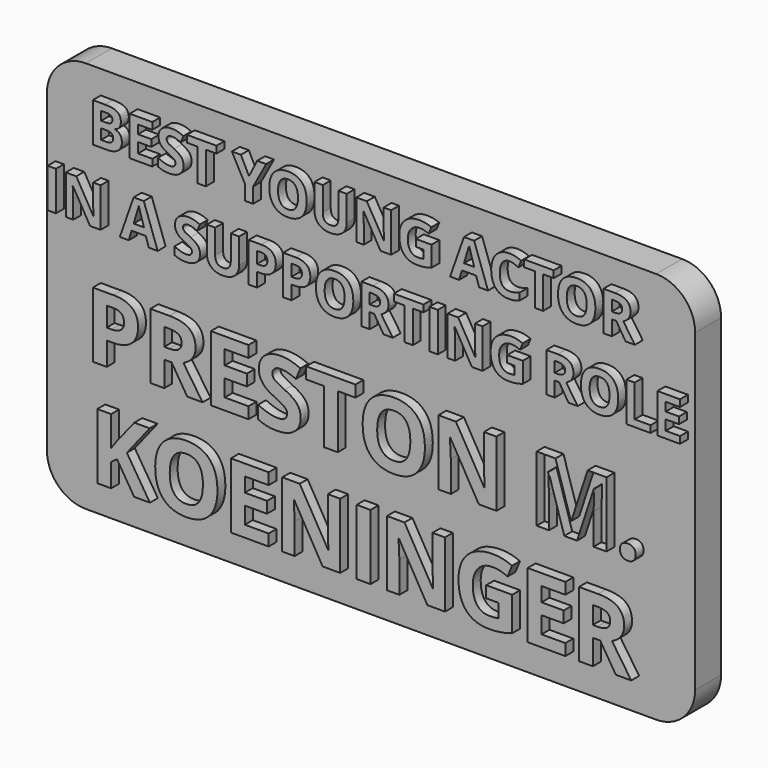
from build123d import *

# Parameters (mm, degrees)
F0_W           = 74
F0_H           = 47
F0_W_2         = 54
F0_H_2         = 27
F0_W_3         = 12.5
F0_H_3         = 6.5
F1_DEPTH       = 12
F2_W           = 54
F2_H           = 27
F3_DEPTH       = 32
F4_W           = 12.5
F4_H           = 6.5
F5_DEPTH       = 1
F7_R           = 3.556
F8_R           = 1.524
F9_R           = 0.762
F10_T          = -2.5
F6_TEXT_SIZE   = 4.2333333333
F6_TEXT_SIZE_2 = 7.0555555556
F11_DEPTH      = 0.762
F12_W          = 81.8964131176
F12_H          = 49.3911341764
F13_DEPTH      = 23.501
F13_DEPTH_BACK = 23.501
F14_W          = 63.7431629002
F14_H          = 29.3685784563
F15_DEPTH      = 30.2390001


# Not quite as in the source:
# - Text() gives the source's letters only with a copy of the font that has no kerning and outlines rounded to 1/6400 em; it was checked with that copy


with BuildPart() as f1:
    # F0 (on Top) → F1 (new body)
    with BuildSketch(Plane.XY):
        Rectangle(F0_W, F0_H)
        Rectangle(F0_W_2, F0_H_2, mode=Mode.SUBTRACT)
        Rectangle(F0_W_2, F0_H_2)
        Rectangle(F0_W_3, F0_H_3, mode=Mode.SUBTRACT)
        Rectangle(F0_W_3, F0_H_3)
    extrude(amount=F1_DEPTH)

    # F2 (on face) → F3 (join)
    with BuildSketch(Plane.XY.offset(12)):
        Rectangle(F2_W, F2_H)
    extrude(amount=F3_DEPTH)

    # F4 (on face) → F5 (cut)
    with BuildSketch(Plane.XY.offset(44)):
        Rectangle(F4_W, F4_H)
    extrude(amount=-F5_DEPTH, mode=Mode.SUBTRACT)

    # F7
    f7_edges = [f1.edges().sort_by_distance(p)[0] for p in [
        (-37, -23.5, 6),
        (37, -23.5, 6),
        (37, 23.5, 6),
        (-37, 23.5, 6),
    ]]
    fillet(f7_edges, radius=F7_R)

    # F8
    f8_edges = [f1.edges().sort_by_distance(p)[0] for p in [
        (-27, -13.5, 28),
        (27, -13.5, 28),
        (27, 13.5, 28),
        (-27, 13.5, 28),
    ]]
    fillet(f8_edges, radius=F8_R)

    # F9
    f9_edges = [f1.edges().sort_by_distance(p)[0] for p in [
        (0, -13.5, 44),
        (0, -23.5, 12),
    ]]
    fillet(f9_edges, radius=F9_R)

    # F10
    f10_openings = [f1.faces().sort_by_distance(p)[0] for p in [
        (0, 0, 0),
    ]]
    offset(amount=F10_T, openings=f10_openings, kind=Kind.INTERSECTION)

    # F6 (on face) → F11 (join)
    with BuildSketch(Plane.XZ.offset(13.5)):
        with Locations((-21.2123072917, 37.904)):
            Text('BEST YOUNG ACTOR', F6_TEXT_SIZE, font='Open Sans', font_style=FontStyle.BOLD, text_align=(TextAlign.LEFT, TextAlign.BOTTOM))
        with Locations((-24.6938932292, 32.316)):
            Text('IN A SUPPORTING ROLE', F6_TEXT_SIZE, font='Open Sans', font_style=FontStyle.BOLD, text_align=(TextAlign.LEFT, TextAlign.BOTTOM))
        with Locations((-21.4571571181, 23.172)):
            Text('PRESTON M.', F6_TEXT_SIZE_2, font='Open Sans', font_style=FontStyle.BOLD, text_align=(TextAlign.LEFT, TextAlign.BOTTOM))
        with Locations((-21.1176085069, 15.044)):
            Text('KOENINGER', F6_TEXT_SIZE_2, font='Open Sans', font_style=FontStyle.BOLD, text_align=(TextAlign.LEFT, TextAlign.BOTTOM))
    extrude(amount=F11_DEPTH)

    # F12 (on Front) → F13 (cut, two sides)
    with BuildSketch(Plane.XZ) as f13_sk:
        with Locations((0.2854410559, 21.6889909934)):
            Rectangle(F12_W, F12_H)
        with BuildLine():
            ThreePointArc((-24.976, 39.738), (-24.0973203436, 41.8593203436), (-21.976, 42.738))
            Line((-21.976, 42.738), (21.976, 42.738))
            ThreePointArc((21.976, 42.738), (24.0973203436, 41.8593203436), (24.976, 39.738))
            Line((24.976, 39.738), (24.976, 15.5))
            ThreePointArc((24.976, 15.5), (24.0973203436, 13.3786796564), (21.976, 12.5))
            Line((21.976, 12.5), (-21.976, 12.5))
            ThreePointArc((-21.976, 12.5), (-24.0973203436, 13.3786796564), (-24.976, 15.5))
            Line((-24.976, 15.5), (-24.976, 39.738))
        make_face(mode=Mode.SUBTRACT)
    extrude(amount=-F13_DEPTH, mode=Mode.SUBTRACT)
    extrude(f13_sk.sketch, amount=F13_DEPTH_BACK, mode=Mode.SUBTRACT)

    # F14 (on face) → F15 (cut, through all)
    with BuildSketch(Plane.XY.offset(42.738)):
        with Locations((-2.1581631154, 3.6842892282)):
            Rectangle(F14_W, F14_H)
    extrude(amount=-F15_DEPTH, mode=Mode.SUBTRACT)


solid = f1.part
